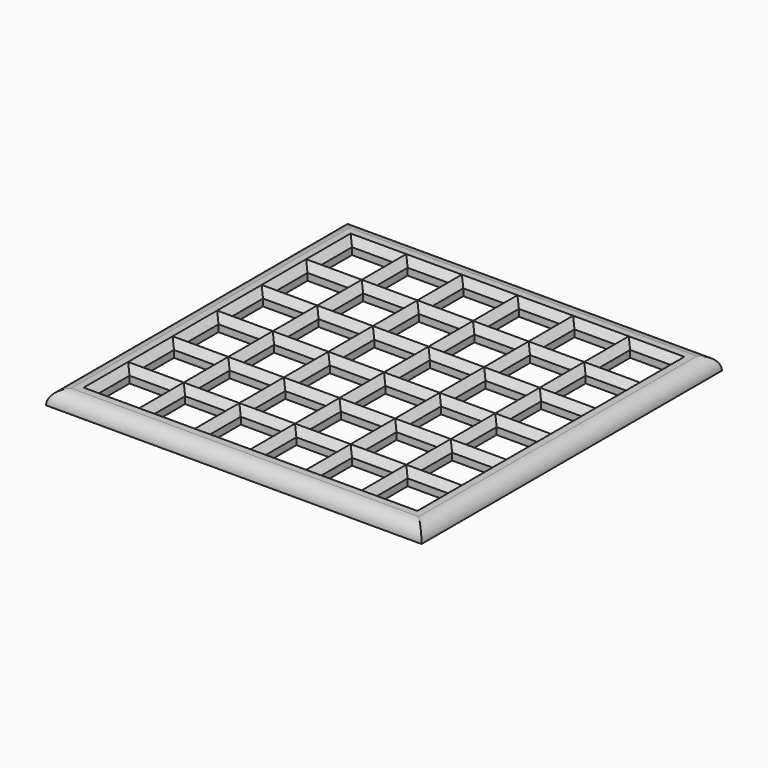
from build123d import *

# Parameters (mm, degrees)
F1_W          = 81
F1_H          = 81
F2_DEPTH      = 3
F0_W          = 9
F0_H          = 9
F3_DEPTH      = 5
F3_DEPTH_BACK = 3
F4_SIZE       = 1.49999
F5_R          = 2.99999


# Not quite as in the source:
# - a fillet or chamfer is up to 0.001 mm smaller than in the source, because OpenCascade refuses the exact size


with BuildPart() as f2:
    # F1 (on Top) → F2 (new body)
    with BuildSketch(Plane.XY):
        with Locations((-34.5, 34.5)):
            Rectangle(F1_W, F1_H)
    extrude(amount=F2_DEPTH)

    # F0 (on Top) → F3 (cut, two sides)
    with BuildSketch(Plane.XY) as f3_sk:
        with Locations((-64.5, 64.5)):
            Rectangle(F0_W, F0_H)
        with Locations((-64.5, 52.5)):
            Rectangle(F0_W, F0_H)
        with Locations((-64.5, 40.5)):
            Rectangle(F0_W, F0_H)
        with Locations((-64.5, 28.5)):
            Rectangle(F0_W, F0_H)
        with Locations((-64.5, 16.5)):
            Rectangle(F0_W, F0_H)
        with Locations((-64.5, 4.5)):
            Rectangle(F0_W, F0_H)
        with Locations((-52.5, 64.5)):
            Rectangle(F0_W, F0_H)
        with Locations((-52.5, 52.5)):
            Rectangle(F0_W, F0_H)
        with Locations((-52.5, 40.5)):
            Rectangle(F0_W, F0_H)
        with Locations((-52.5, 28.5)):
            Rectangle(F0_W, F0_H)
        with Locations((-52.5, 16.5)):
            Rectangle(F0_W, F0_H)
        with Locations((-52.5, 4.5)):
            Rectangle(F0_W, F0_H)
        with Locations((-40.5, 64.5)):
            Rectangle(F0_W, F0_H)
        with Locations((-40.5, 52.5)):
            Rectangle(F0_W, F0_H)
        with Locations((-40.5, 40.5)):
            Rectangle(F0_W, F0_H)
        with Locations((-40.5, 28.5)):
            Rectangle(F0_W, F0_H)
        with Locations((-40.5, 16.5)):
            Rectangle(F0_W, F0_H)
        with Locations((-40.5, 4.5)):
            Rectangle(F0_W, F0_H)
        with Locations((-28.5, 64.5)):
            Rectangle(F0_W, F0_H)
        with Locations((-28.5, 52.5)):
            Rectangle(F0_W, F0_H)
        with Locations((-28.5, 40.5)):
            Rectangle(F0_W, F0_H)
        with Locations((-28.5, 28.5)):
            Rectangle(F0_W, F0_H)
        with Locations((-28.5, 16.5)):
            Rectangle(F0_W, F0_H)
        with Locations((-28.5, 4.5)):
            Rectangle(F0_W, F0_H)
        with Locations((-16.5, 64.5)):
            Rectangle(F0_W, F0_H)
        with Locations((-16.5, 52.5)):
            Rectangle(F0_W, F0_H)
        with Locations((-16.5, 40.5)):
            Rectangle(F0_W, F0_H)
        with Locations((-16.5, 28.5)):
            Rectangle(F0_W, F0_H)
        with Locations((-16.5, 16.5)):
            Rectangle(F0_W, F0_H)
        with Locations((-16.5, 4.5)):
            Rectangle(F0_W, F0_H)
        with Locations((-4.5, 64.5)):
            Rectangle(F0_W, F0_H)
        with Locations((-4.5, 52.5)):
            Rectangle(F0_W, F0_H)
        with Locations((-4.5, 40.5)):
            Rectangle(F0_W, F0_H)
        with Locations((-4.5, 28.5)):
            Rectangle(F0_W, F0_H)
        with Locations((-4.5, 16.5)):
            Rectangle(F0_W, F0_H)
        with Locations((-4.5, 4.5)):
            Rectangle(F0_W, F0_H)
    extrude(amount=F3_DEPTH, mode=Mode.SUBTRACT)
    extrude(f3_sk.sketch, amount=-F3_DEPTH_BACK, mode=Mode.SUBTRACT)

    # F4 (size 1.5 in the source; OpenCascade refuses exactly that, so slightly less here)
    f4_edges = [f2.edges().sort_by_distance(p)[0] for p in [
        (-64.5, 69, 3),
        (-69, 64.5, 3),
        (-60, 64.5, 3),
        (-64.5, 60, 3),
        (-52.5, 69, 3),
        (-57, 64.5, 3),
        (-52.5, 60, 3),
        (-48, 64.5, 3),
        (-45, 64.5, 3),
        (-36, 64.5, 3),
        (-33, 64.5, 3),
        (-24, 64.5, 3),
        (-21, 64.5, 3),
        (-12, 64.5, 3),
        (-9, 64.5, 3),
        (0, 64.5, 3),
        (-69, 52.5, 3),
        (-60, 52.5, 3),
        (-57, 52.5, 3),
        (-48, 52.5, 3),
        (-45, 52.5, 3),
        (-36, 52.5, 3),
        (-33, 52.5, 3),
        (-24, 52.5, 3),
        (-21, 52.5, 3),
        (-12, 52.5, 3),
        (-9, 52.5, 3),
        (0, 52.5, 3),
        (-69, 40.5, 3),
        (-60, 40.5, 3),
        (-57, 40.5, 3),
        (-48, 40.5, 3),
        (-45, 40.5, 3),
        (-36, 40.5, 3),
        (-33, 40.5, 3),
        (-24, 40.5, 3),
        (-21, 40.5, 3),
        (-12, 40.5, 3),
        (-9, 40.5, 3),
        (0, 40.5, 3),
        (-69, 28.5, 3),
        (-60, 28.5, 3),
        (-57, 28.5, 3),
        (-48, 28.5, 3),
        (-45, 28.5, 3),
        (-36, 28.5, 3),
        (-33, 28.5, 3),
        (-24, 28.5, 3),
        (-21, 28.5, 3),
        (-12, 28.5, 3),
        (-9, 28.5, 3),
        (0, 28.5, 3),
        (0, 16.5, 3),
        (-9, 16.5, 3),
        (-12, 16.5, 3),
        (-21, 16.5, 3),
        (-24, 16.5, 3),
        (-33, 16.5, 3),
        (-45, 16.5, 3),
        (-48, 16.5, 3),
        (-57, 16.5, 3),
        (-60, 16.5, 3),
        (-69, 16.5, 3),
        (-69, 4.5, 3),
        (-60, 4.5, 3),
        (-57, 4.5, 3),
        (-48, 4.5, 3),
        (-45, 4.5, 3),
        (-36, 4.5, 3),
        (-33, 4.5, 3),
        (-24, 4.5, 3),
        (-21, 4.5, 3),
        (-12, 4.5, 3),
        (-9, 4.5, 3),
        (0, 4.5, 3),
        (-36, 16.5, 3),
        (-4.5, 9, 3),
        (-16.5, 9, 3),
        (-28.5, 9, 3),
        (-40.5, 9, 3),
        (-52.5, 9, 3),
        (-64.5, 9, 3),
        (-64.5, 0, 3),
        (-52.5, 0, 3),
        (-40.5, 0, 3),
        (-28.5, 0, 3),
        (-16.5, 0, 3),
        (-4.5, 0, 3),
        (-4.5, 21, 3),
        (-16.5, 21, 3),
        (-28.5, 21, 3),
        (-40.5, 21, 3),
        (-52.5, 21, 3),
        (-64.5, 21, 3),
        (-64.5, 33, 3),
        (-52.5, 33, 3),
        (-40.5, 33, 3),
        (-28.5, 33, 3),
        (-16.5, 33, 3),
        (-4.5, 33, 3),
        (-4.5, 45, 3),
        (-16.5, 45, 3),
        (-28.5, 45, 3),
        (-40.5, 45, 3),
        (-52.5, 45, 3),
        (-64.5, 45, 3),
        (-64.5, 57, 3),
        (-52.5, 57, 3),
        (-40.5, 57, 3),
        (-28.5, 57, 3),
        (-16.5, 57, 3),
        (-4.5, 57, 3),
        (-4.5, 69, 3),
        (-16.5, 69, 3),
        (-28.5, 69, 3),
        (-40.5, 69, 3),
        (-64.5, 12, 3),
        (-52.5, 12, 3),
        (-40.5, 12, 3),
        (-28.5, 12, 3),
        (-16.5, 12, 3),
        (-4.5, 12, 3),
        (-4.5, 24, 3),
        (-16.5, 24, 3),
        (-28.5, 24, 3),
        (-40.5, 24, 3),
        (-52.5, 24, 3),
        (-64.5, 24, 3),
        (-64.5, 36, 3),
        (-52.5, 36, 3),
        (-40.5, 36, 3),
        (-28.5, 36, 3),
        (-16.5, 36, 3),
        (-4.5, 36, 3),
        (-4.5, 48, 3),
        (-16.5, 48, 3),
        (-28.5, 48, 3),
        (-40.5, 48, 3),
        (-52.5, 48, 3),
        (-64.5, 48, 3),
        (-4.5, 60, 3),
        (-16.5, 60, 3),
        (-28.5, 60, 3),
        (-40.5, 60, 3),
    ]]
    chamfer(f4_edges, length=F4_SIZE)

    # F5 (radius 3 in the source; OpenCascade refuses exactly that, so slightly less here)
    f5_edges = [f2.edges().sort_by_distance(p)[0] for p in [
        (-34.5, 75, 3),
        (-75, 34.5, 3),
        (-34.5, -6, 3),
        (6, 34.5, 3),
    ]]
    fillet(f5_edges, radius=F5_R)


solid = f2.part
